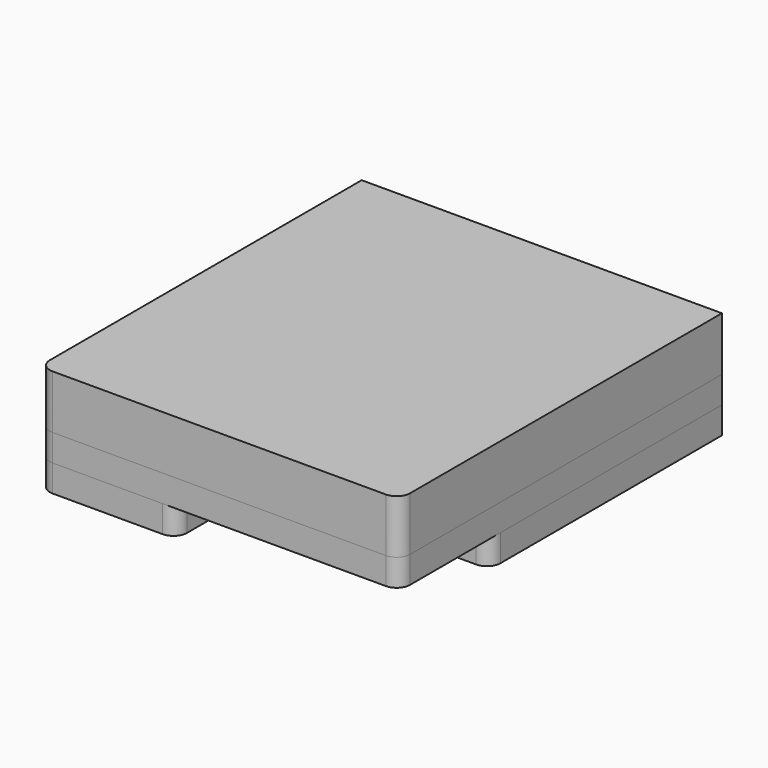
from build123d import *

# Parameters (mm, degrees)
F0_W      = 85.09
F0_H      = 95.25
F1_DEPTH  = 6.35
F2_R      = 1.905
F2_W      = 6.35
F2_H      = 12.7
F2_H_2    = 6.35
F2_H_3    = 25.4
F2_W_2    = 27.94
F2_H_4    = 13.97
F3_DEPTH  = 6.351
F4_DEPTH  = 133
F5_DEPTH  = 6.35
F6_W      = 52.705
F6_H      = 26.67
F6_W_2    = 6.35
F6_H_2    = 12.7
F7_DEPTH  = 6.35
F8_R      = 3.175
F8_2_R    = 3.175
F10_DEPTH = 12.7


# Not quite as in the source:
# - an extrude ends at something that could not be found from the text; its depth is read off the source's solid


with BuildPart() as f1:
    # F0 (on Top) → F1 (new body)
    with BuildSketch(Plane.XY):
        Rectangle(F0_W, F0_H)
    extrude(amount=F1_DEPTH)

    # F2 (on Top) → F3 (cut, through all)
    with BuildSketch(Plane.XY):
        with Locations((-23.495, -32.385)):
            Circle(F2_R)
        with Locations((-23.495, 18.415)):
            Circle(F2_R)
        with Locations((1.905, -32.385)):
            Rectangle(F2_W, F2_H)
        with Locations((1.905, 27.94)):
            Rectangle(F2_W, F2_H_2)
        with Locations((1.905, 18.415)):
            Rectangle(F2_W, F2_H)
        with Locations((1.905, 8.89)):
            Rectangle(F2_W, F2_H_2)
        with Locations((20.955, 18.415)):
            Rectangle(F2_W, F2_H)
        with Locations((20.955, 27.94)):
            Rectangle(F2_W, F2_H_2)
        with Locations((20.955, 8.89)):
            Rectangle(F2_W, F2_H_2)
        with Locations((20.955, -32.385)):
            Rectangle(F2_W, F2_H)
        with Locations((11.43, 27.94)):
            Rectangle(F2_W, F2_H_2)
        with Locations((11.43, 18.415)):
            Rectangle(F2_W, F2_H)
        with Locations((11.43, 8.89)):
            Rectangle(F2_W, F2_H_2)
        with Locations((11.43, -32.385)):
            Rectangle(F2_W, F2_H)
        with Locations((30.48, -32.385)):
            Rectangle(F2_W, F2_H)
        with Locations((30.48, 18.415)):
            Rectangle(F2_W, F2_H_3)
        with Locations((16.1925, -10.16)):
            Rectangle(F2_W_2, F2_H_4)
        with Locations((-23.495, -10.16)):
            Circle(F2_R)
        with Locations((-36.195, -10.16)):
            Circle(F2_R)
        with Locations((-10.795, -10.16)):
            Circle(F2_R)
        with Locations((-31.75, 40.005)):
            Circle(F2_R)
        with Locations((-15.875, 40.005)):
            Circle(F2_R)
        with Locations((0, 40.005)):
            Circle(F2_R)
        with Locations((15.875, 40.005)):
            Circle(F2_R)
        with Locations((31.75, 40.005)):
            Circle(F2_R)
    extrude(amount=F3_DEPTH, mode=Mode.SUBTRACT)

    # F2 (on Top) → F4 (cut, through all)
    with BuildSketch(Plane.XY):
        with Locations((-23.495, -32.385)):
            Circle(F2_R)
        with Locations((-23.495, 18.415)):
            Circle(F2_R)
        with Locations((1.905, -32.385)):
            Rectangle(F2_W, F2_H)
        with Locations((1.905, 27.94)):
            Rectangle(F2_W, F2_H_2)
        with Locations((1.905, 18.415)):
            Rectangle(F2_W, F2_H)
        with Locations((1.905, 8.89)):
            Rectangle(F2_W, F2_H_2)
        with Locations((20.955, 18.415)):
            Rectangle(F2_W, F2_H)
        with Locations((20.955, 27.94)):
            Rectangle(F2_W, F2_H_2)
        with Locations((20.955, 8.89)):
            Rectangle(F2_W, F2_H_2)
        with Locations((20.955, -32.385)):
            Rectangle(F2_W, F2_H)
        with Locations((11.43, 27.94)):
            Rectangle(F2_W, F2_H_2)
        with Locations((11.43, 18.415)):
            Rectangle(F2_W, F2_H)
        with Locations((11.43, 8.89)):
            Rectangle(F2_W, F2_H_2)
        with Locations((11.43, -32.385)):
            Rectangle(F2_W, F2_H)
        with Locations((30.48, -32.385)):
            Rectangle(F2_W, F2_H)
        with Locations((30.48, 18.415)):
            Rectangle(F2_W, F2_H_3)
        with Locations((16.1925, -10.16)):
            Rectangle(F2_W_2, F2_H_4)
        with Locations((-23.495, -10.16)):
            Circle(F2_R)
        with Locations((-36.195, -10.16)):
            Circle(F2_R)
        with Locations((-10.795, -10.16)):
            Circle(F2_R)
        with Locations((-31.75, 40.005)):
            Circle(F2_R)
        with Locations((-15.875, 40.005)):
            Circle(F2_R)
        with Locations((0, 40.005)):
            Circle(F2_R)
        with Locations((15.875, 40.005)):
            Circle(F2_R)
        with Locations((31.75, 40.005)):
            Circle(F2_R)
    extrude(amount=-F4_DEPTH, mode=Mode.SUBTRACT)


with BuildPart() as f5:
    # F5 (new): a face of the model
    f5_faces = [f1.part.faces().sort_by_distance(p)[0] for p in [
        (-3.113503162, 0.1142969889, 0),
    ]]
    extrude(f5_faces, amount=F5_DEPTH)

    # F6 (on face) → F7 (cut, through all)
    with BuildSketch(Plane(origin=(0, 0, -6.35), x_dir=(1, 0, 0), z_dir=(0, 0, -1))):
        with Locations((16.1925, 34.29)):
            Rectangle(F6_W, F6_H)
        with Locations((1.905, 32.385)):
            Rectangle(F6_W_2, F6_H_2, mode=Mode.SUBTRACT)
        with Locations((11.43, 32.385)):
            Rectangle(F6_W_2, F6_H_2, mode=Mode.SUBTRACT)
        with Locations((20.955, 32.385)):
            Rectangle(F6_W_2, F6_H_2, mode=Mode.SUBTRACT)
        with Locations((30.48, 32.385)):
            Rectangle(F6_W_2, F6_H_2, mode=Mode.SUBTRACT)
    extrude(amount=-F7_DEPTH, mode=Mode.SUBTRACT)

    # F8#2
    f8_2_edges = [f5.edges().sort_by_distance(p)[0] for p in [
        (-10.16, -47.625, -3.175),
        (-10.16, -20.955, -3.175),
        (42.545, -20.955, -3.175),
        (-42.545, -47.625, -3.175),
    ]]
    fillet(f8_2_edges, radius=F8_2_R)


with BuildPart() as f1_1:
    add(f1.part)

    # F8
    f8_edges = [f1_1.edges().sort_by_distance(p)[0] for p in [
        (42.545, -47.625, 3.175),
        (-42.545, -47.625, 3.175),
    ]]
    fillet(f8_edges, radius=F8_R)


with BuildPart() as f10:
    # F9 (on face) → F10 (new body)
    with BuildSketch(Plane.XY.offset(6.35)):
        with BuildLine():
            Line((42.545, 47.625), (-42.545, 47.625))
            Line((-42.545, 47.625), (-42.545, -44.45))
            ThreePointArc((-42.545, -44.45), (-41.6150640303, -46.6950640303), (-39.37, -47.625))
            Line((-39.37, -47.625), (39.37, -47.625))
            ThreePointArc((39.37, -47.625), (41.6150640303, -46.6950640303), (42.545, -44.45))
            Line((42.545, -44.45), (42.545, 47.625))
        make_face()
    extrude(amount=F10_DEPTH)


solid = Compound([f5.part, f1_1.part, f10.part])
